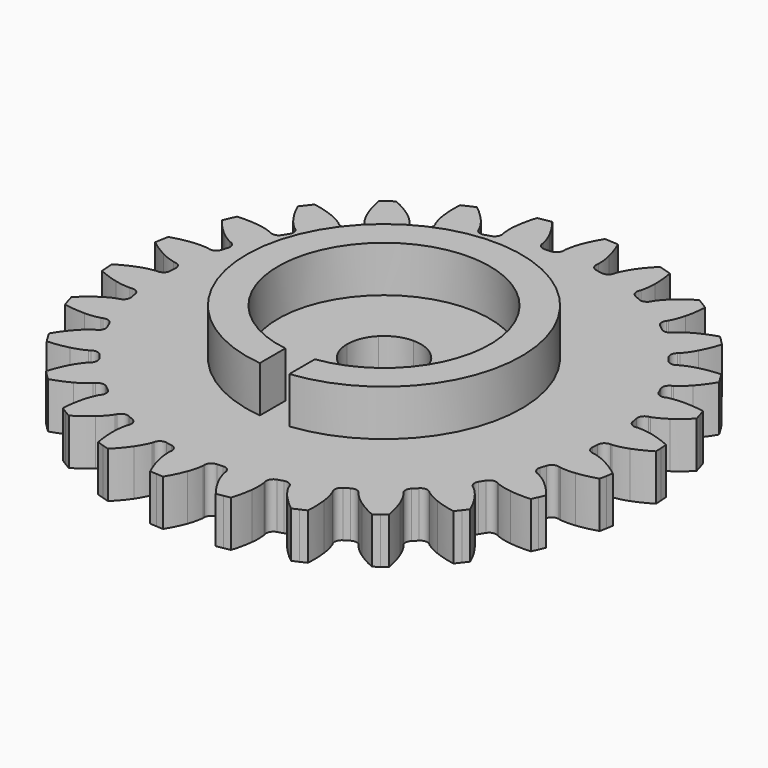
from build123d import *

# Parameters (mm, degrees)
F1_R            = 24.0875
F2_DEPTH        = 5
F4_DEPTH        = 5.001
F6_DEPTH        = 5
F6_COPIES_COUNT = 26
F7_R            = 14.9091518161
F7_R_2          = 11.4755582031
F8_DEPTH        = 5
F10_DEPTH       = 5


# Not quite as in the source:
# - a pattern or mirror of a feature is missing from the dataset's text; its kind, count and spacing are read off the source's solid


with BuildPart() as f2:
    # F1 (on Top) → F2 (new body)
    with BuildSketch(Plane.XY):
        Circle(F1_R)
    extrude(amount=F2_DEPTH)

    # F3 (on face) → F4 (cut, through all)
    with BuildSketch(Plane.XY.offset(5)):
        with BuildLine():
            ThreePointArc((0, 4), (-1.5491933385, 3.6878177829), (-2.8565713714, 2.8))
            ThreePointArc((-2.8565713714, 2.8), (-3.7031260771, 1.5122358471), (-4, 0))
            ThreePointArc((-4, 0), (1.5122358471, -3.7031260771), (2.8565713714, 2.8))
            ThreePointArc((2.8565713714, 2.8), (1.5491933385, 3.6878177829), (0, 4))
        make_face()
    extrude(amount=-F4_DEPTH, mode=Mode.SUBTRACT)

    # F5 (on Top) → F6 (join)
    with BuildSketch(Plane.XY):
        with BuildLine():
            ThreePointArc((1.7339174542, 28.6475745965), (1.36734888, 28.6674093186), (1.0005565906, 28.6825536957))
            ThreePointArc((1.0005565906, 28.6825536957), (0.4512361223, 27.6904186304), (0, 26.65))
            ThreePointArc((0, 26.65), (1.6100662075, 26.6013192682), (3.2142502986, 26.4554549199))
            ThreePointArc((3.2142502986, 26.4554549199), (2.8917928502, 27.5427019749), (2.4661436024, 28.5938478651))
            ThreePointArc((2.4661436024, 28.5938478651), (2.1002023379, 28.6230527746), (1.7339174542, 28.6475745965))
        make_face()
        with BuildLine():
            ThreePointArc((3.2142502986, 26.4554549199), (1.6100662075, 26.6013192682), (0, 26.65))
            ThreePointArc((0, 26.65), (-0.2476347728, 25.8567199837), (-0.3992066379, 25.0396262714))
            Line((-0.3992066379, 25.0396262714), (-0.3960547586, 24.8419294617))
            ThreePointArc((-0.3960547586, 24.8419294617), (-0.6045120787, 24.3029076621), (-1.1293778433, 24.0610091629))
            ThreePointArc((-1.1293778433, 24.0610091629), (1.4552521491, 24.0435001078), (4.0231260978, 23.7491497248))
            ThreePointArc((4.0231260978, 23.7491497248), (3.5312671766, 24.052586302), (3.3893428894, 24.6128152296))
            Line((3.3893428894, 24.6128152296), (3.4163159261, 24.8086887047))
            ThreePointArc((3.4163159261, 24.8086887047), (3.3644000186, 25.6380986778), (3.2142502986, 26.4554549199))
        make_face()
    f6 = extrude(amount=F6_DEPTH)

    # F6_copies: F6 ×26 about axis
    f6_copies_axis = Axis((0, 0, 0), (0, 0, 1))
    for i in range(1, F6_COPIES_COUNT):
        add(f6.rotate(f6_copies_axis, i * 360 / F6_COPIES_COUNT))

    # F7 (on face) → F8 (join)
    with BuildSketch(Plane.XY.offset(5)):
        Circle(F7_R)
        Circle(F7_R_2, mode=Mode.SUBTRACT)
    extrude(amount=F8_DEPTH)

    # F9 (on face) → F10 (cut)
    with BuildSketch(Plane.XY.offset(10)):
        with BuildLine():
            Line((1.6, -13.0932596261), (0, -13.0932596261))
            Line((0, -13.0932596261), (0, -14.9091518161))
            ThreePointArc((0, -14.9091518161), (0.8011575286, -14.8876107717), (1.6, -14.8230498844))
            Line((1.6, -14.8230498844), (1.6, -13.0932596261))
        make_face()
        with BuildLine():
            ThreePointArc((1.6, -11.3634693678), (0.8019607077, -11.4475016967), (0, -11.4755582031))
            Line((0, -11.4755582031), (0, -13.0932596261))
            Line((0, -13.0932596261), (1.6, -13.0932596261))
            Line((1.6, -13.0932596261), (1.6, -11.3634693678))
        make_face()
        with BuildLine():
            Line((0, -14.9091518161), (0, -13.0932596261))
            Line((0, -13.0932596261), (-1.6, -13.0932596261))
            Line((-1.6, -13.0932596261), (-1.6, -14.8230498844))
            ThreePointArc((-1.6, -14.8230498844), (-0.8011575286, -14.8876107717), (0, -14.9091518161))
        make_face()
        with BuildLine():
            Line((0, -13.0932596261), (0, -11.4755582031))
            ThreePointArc((0, -11.4755582031), (-0.8019607077, -11.4475016967), (-1.6, -11.3634693678))
            Line((-1.6, -11.3634693678), (-1.6, -13.0932596261))
            Line((-1.6, -13.0932596261), (0, -13.0932596261))
        make_face()
    extrude(amount=-F10_DEPTH, mode=Mode.SUBTRACT)


solid = f2.part
